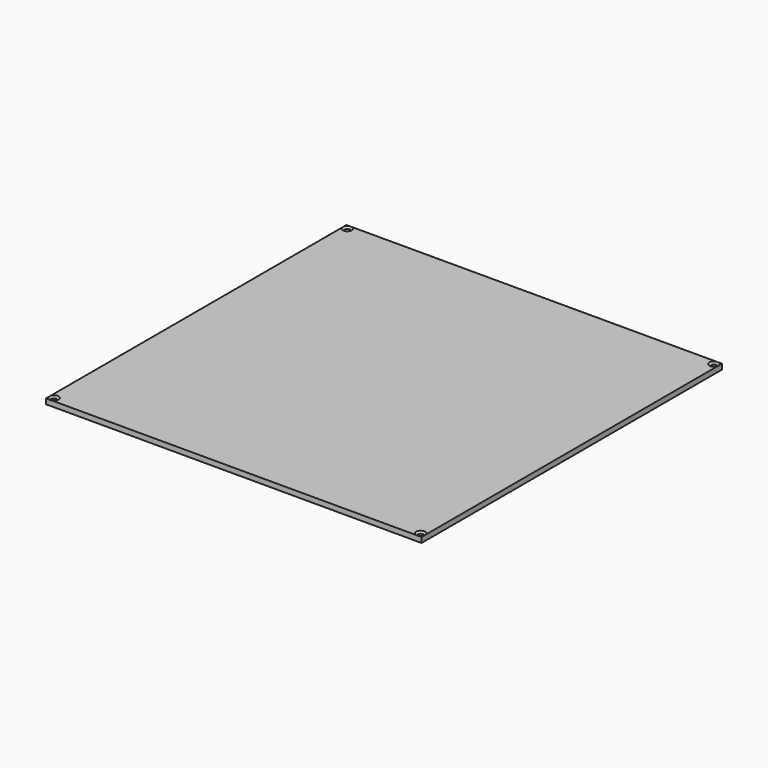
from build123d import *

# Parameters (mm, degrees)
F0_R     = 1.6
F1_DEPTH = 3


# Not quite as in the source:
# - a fillet or chamfer that OpenCascade refuses, or shapes differently, is made with other operations: its cross-section is extruded or revolved along the edge and cut away or added


with BuildPart() as f1:
    # F0 (on Top) → F1 (new body)
    with BuildSketch(Plane.XY):
        Polygon((-107, 107), (-107, 0), (-107, -107), (0, -107), (107, -107), (107, 0), (107, 107), (0, 107), align=None)
        with Locations((-104.5, -104.5)):
            Circle(F0_R, mode=Mode.SUBTRACT)
        with Locations((104.5, -104.5)):
            Circle(F0_R, mode=Mode.SUBTRACT)
        with Locations((-104.5, 104.5)):
            Circle(F0_R, mode=Mode.SUBTRACT)
        with Locations((104.5, 104.5)):
            Circle(F0_R, mode=Mode.SUBTRACT)
    extrude(amount=F1_DEPTH)

    # F2: chamfer of 1 on 4 edges, made by hand

    # F2_s1 → F2_t2 (revolve, cut)
    with BuildSketch(Plane.XZ.offset(104.5)):
        Polygon((-102.9, 2), (-101.9, 3), (-102.9, 3), align=None)
    revolve(axis=Axis((-104.5, -104.5, 3), (0, 0, 1)), mode=Mode.SUBTRACT)

    # F2_s3 → F2_t4 (revolve, cut)
    with BuildSketch(Plane.XZ.offset(-104.5)):
        Polygon((-102.9, 2), (-101.9, 3), (-102.9, 3), align=None)
    revolve(axis=Axis((-104.5, 104.5, 3), (0, 0, 1)), mode=Mode.SUBTRACT)

    # F2_s5 → F2_t6 (revolve, cut)
    with BuildSketch(Plane.XZ.offset(-104.5)):
        Polygon((106.1, 2), (107.1, 3), (106.1, 3), align=None)
    revolve(axis=Axis((104.5, 104.5, 3), (0, 0, 1)), mode=Mode.SUBTRACT)

    # F2_s7 → F2_t8 (revolve, cut)
    with BuildSketch(Plane.XZ.offset(104.5)):
        Polygon((106.1, 2), (107.1, 3), (106.1, 3), align=None)
    revolve(axis=Axis((104.5, -104.5, 3), (0, 0, 1)), mode=Mode.SUBTRACT)


solid = f1.part
